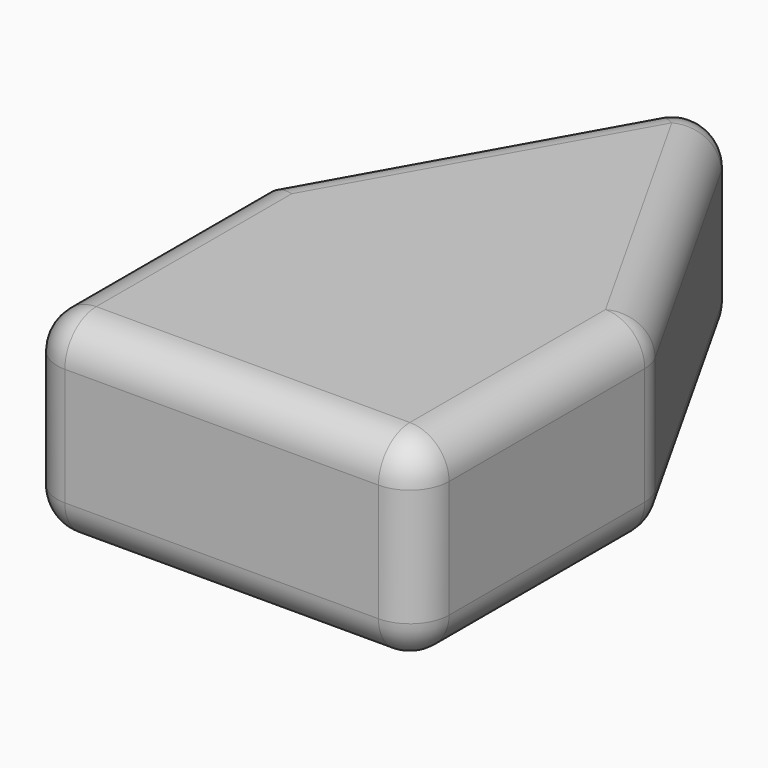
from build123d import *

# Parameters (mm, degrees)
F0_W     = 20
F0_H     = 15
F1_DEPTH = 10
F3_R     = 2


# Not quite as in the source:
# - a feature of the source that left no trace in its solid (it failed there, or was rolled back) is left out


with BuildPart() as f1:
    # F0 (on Top) → F1 (new body)
    with BuildSketch(Plane.XY):
        Polygon((0, 24.5688632738), (-10, 6.7879746571), (10, 6.7879746571), align=None)
        with Locations((0, -0.7120253429)):
            Rectangle(F0_W, F0_H)
    extrude(amount=F1_DEPTH)

    # F3
    f3_edges = [f1.edges().sort_by_distance(p)[0] for p in [
        (-10, -0.712025, 0),
        (-5, 15.678419, 0),
        (0, 24.568863, 5),
        (-5, 15.678419, 10),
        (-10, -8.212025, 5),
        (-10, -0.712025, 10),
        (10, -8.212025, 5),
        (0, -8.212025, 0),
        (0, -8.212025, 10),
        (10, 6.787975, 5),
        (10, -0.712025, 0),
        (10, -0.712025, 10),
        (5, 15.678419, 0),
        (5, 15.678419, 10),
    ]]
    fillet(f3_edges, radius=F3_R)


solid = f1.part
